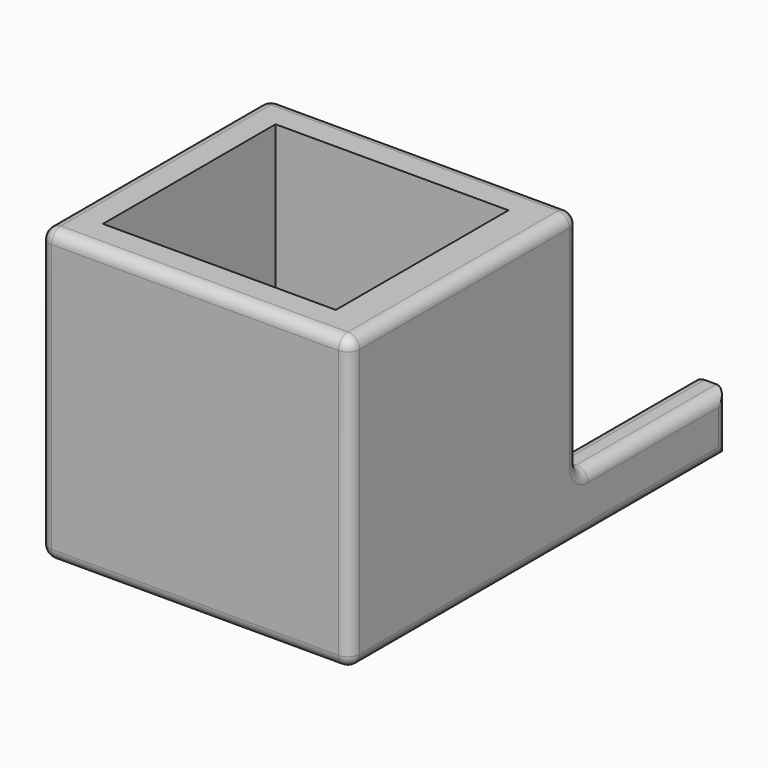
from build123d import *

# Parameters (mm, degrees)
F1_DEPTH = 25
F2_W     = 16
F2_H     = 20
F3_DEPTH = 26.601
F4_W     = 19.9722627059
F4_H     = 18.5
F5_DEPTH = 25.001
F6_R     = 1


with BuildPart() as f1:
    # F0 (on Top) → F1 (new body)
    with BuildSketch(Plane.XY):
        Polygon((-13.3, 40.5), (-13.3, 0), (0, 0), (13.3, 0), (13.3, 40.5), (10.3, 40.5), (10.3, 24.5), (0, 24.5), (-10.3, 24.5), (-10.3, 40.5), align=None)
    extrude(amount=F1_DEPTH)

    # F2 (on face) → F3 (cut, through all)
    with BuildSketch(Plane(origin=(-13.3, 0, 0), x_dir=(0, -1, 0), z_dir=(-1, 0, 0))):
        with Locations((-32.5, 15)):
            Rectangle(F2_W, F2_H)
    extrude(amount=-F3_DEPTH, mode=Mode.SUBTRACT)

    # F4 (on face) → F5 (cut, through all)
    with BuildSketch(Plane.XY):
        with Locations((-0.3138686471, 12.25)):
            Rectangle(F4_W, F4_H)
    extrude(amount=F5_DEPTH, mode=Mode.SUBTRACT)

    # F6
    f6_edges = [f1.edges().sort_by_distance(p)[0] for p in [
        (13.3, 20.25, 0),
        (13.3, 40.5, 2.5),
        (13.3, 32.5, 5),
        (13.3, 24.5, 15),
        (13.3, 12.25, 25),
        (13.3, 0, 12.5),
        (-13.3, 20.25, 0),
        (-13.3, 0, 12.5),
        (-13.3, 12.25, 25),
        (-13.3, 24.5, 15),
        (-13.3, 32.5, 5),
        (-13.3, 40.5, 2.5),
        (0, 0, 25),
        (0, 0, 0),
        (0, 24.5, 25),
        (0, 24.5, 0),
        (-11.8, 24.5, 5),
        (11.8, 24.5, 5),
        (10.3, 32.5, 5),
        (-10.3, 32.5, 0),
        (-10.3, 40.5, 2.5),
        (-10.3, 32.5, 5),
        (-10.3, 24.5, 2.5),
        (10.3, 32.5, 0),
        (10.3, 24.5, 2.5),
    ]]
    fillet(f6_edges, radius=F6_R)


solid = f1.part
